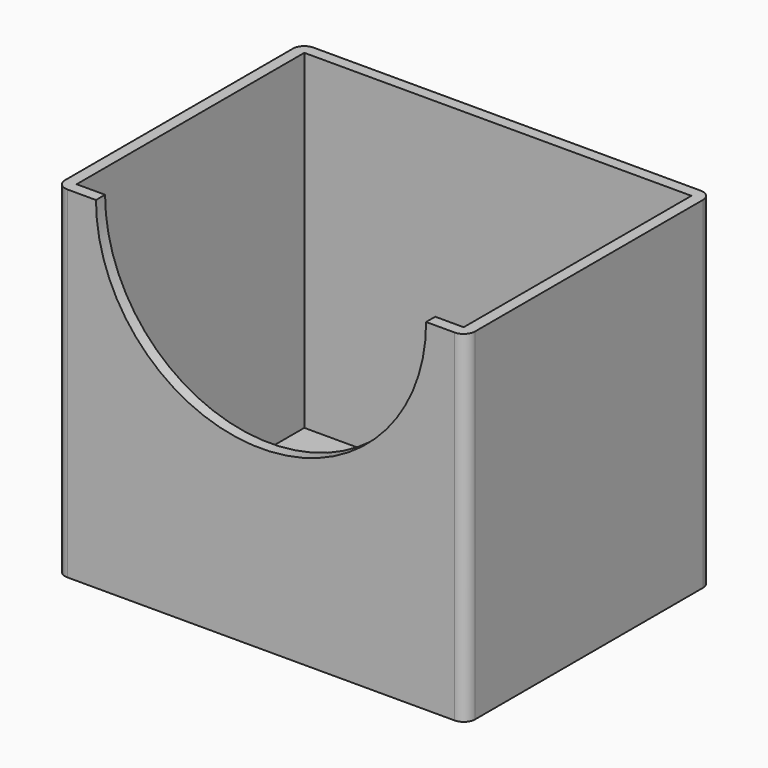
from build123d import *

# Parameters (mm, degrees)
F0_W     = 68
F0_H     = 50
F1_DEPTH = 2
F0_W_2   = 72
F0_H_2   = 54
F2_DEPTH = 60
F4_DEPTH = 25
F5_R     = 2


# Not quite as in the source:
# - a feature names something its author has since deleted; it is built from what else it names


with BuildPart() as f1:
    # F0 (on Top) → F1 (new body)
    with BuildSketch(Plane.XY):
        Rectangle(F0_W, F0_H)
    extrude(amount=F1_DEPTH)

    # F0 (on Top) → F2 (join)
    with BuildSketch(Plane.XY):
        Rectangle(F0_W_2, F0_H_2)
        Rectangle(F0_W, F0_H, mode=Mode.SUBTRACT)
    extrude(amount=F2_DEPTH)

    # F3 (on face) → F4 (cut)
    with BuildSketch(Plane(origin=(0, -25, 0), x_dir=(-1, 0, 0), z_dir=(0, 1, 0))):
        with BuildLine():
            Line((29, 60), (-29, 60))
            ThreePointArc((-29, 60), (0, 31), (29, 60))
        make_face()
    extrude(amount=-F4_DEPTH, mode=Mode.SUBTRACT)

    # F5
    f5_edges = [f1.edges().sort_by_distance(p)[0] for p in [
        (-36, 27, 30),
        (36, 27, 30),
        (-36, -27, 30),
        (36, -27, 30),
    ]]
    fillet(f5_edges, radius=F5_R)


solid = f1.part
